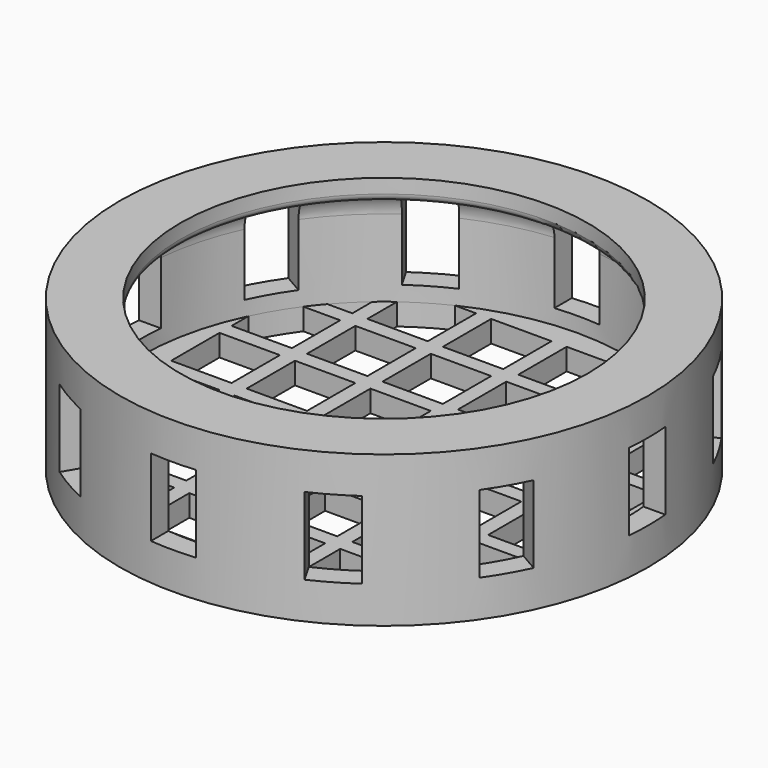
from build123d import *

# Parameters (mm, degrees)
F2_W            = 4
F2_H            = 4
F3_DEPTH        = 1.44
F4_R            = 17.5
F4_R_2          = 16.06
F5_DEPTH        = 1.44
F6_W            = 4
F6_H            = 5.12
F7_DEPTH        = 1.5
F7_COPIES_COUNT = 12


# Not quite as in the source:
# - a pattern or mirror of a feature is missing from the dataset's text; its kind, count and spacing are read off the source's solid


with BuildPart() as f1:
    # F0 (on Front) → F1 (revolve)
    with BuildSketch(Plane.XZ):
        with BuildLine():
            Line((0, 1.44), (0, 0))
            Line((0, 0), (17.5, 0))
            Line((17.5, 0), (17.5, 10))
            Line((17.5, 10), (13.5, 10))
            Line((13.5, 10), (13.5, 9.06))
            ThreePointArc((13.5, 9.06), (13.6464466094, 8.7064466094), (14, 8.56))
            Line((14, 8.56), (14.06, 8.56))
            ThreePointArc((14.06, 8.56), (15.4742135624, 7.9742135624), (16.06, 6.56))
            Line((16.06, 6.56), (16.06, 1.44))
            Line((16.06, 1.44), (0, 1.44))
        make_face()
    revolve(axis=Axis((0, 0, 0.72), (0, 0, 1)))

    # F2 (on face) → F3 (cut, through all)
    with BuildSketch(Plane(origin=(0, 0, 0), x_dir=(1, 0, 0), z_dir=(0, 0, -1))):
        with Locations((2.5, 2.5)):
            Rectangle(F2_W, F2_H)
        with Locations((2.5, 7.5)):
            Rectangle(F2_W, F2_H)
        with Locations((2.5, 12.5)):
            Rectangle(F2_W, F2_H)
        with Locations((7.5, 2.5)):
            Rectangle(F2_W, F2_H)
        with Locations((7.5, 7.5)):
            Rectangle(F2_W, F2_H)
        with Locations((7.5, 12.5)):
            Rectangle(F2_W, F2_H)
        with Locations((12.5, 2.5)):
            Rectangle(F2_W, F2_H)
        with Locations((12.5, 7.5)):
            Rectangle(F2_W, F2_H)
        with Locations((12.5, 12.5)):
            Rectangle(F2_W, F2_H)
        with Locations((-12.5, 2.5)):
            Rectangle(F2_W, F2_H)
        with Locations((-2.5, 2.5)):
            Rectangle(F2_W, F2_H)
        with Locations((-7.5, 7.5)):
            Rectangle(F2_W, F2_H)
        with Locations((-7.5, 12.5)):
            Rectangle(F2_W, F2_H)
        with Locations((-12.5, 7.5)):
            Rectangle(F2_W, F2_H)
        with Locations((-7.5, 2.5)):
            Rectangle(F2_W, F2_H)
        with Locations((-12.5, 12.5)):
            Rectangle(F2_W, F2_H)
        with Locations((-2.5, 7.5)):
            Rectangle(F2_W, F2_H)
        with Locations((-2.5, 12.5)):
            Rectangle(F2_W, F2_H)
        with Locations((2.5, -2.5)):
            Rectangle(F2_W, F2_H)
        with Locations((12.5, -2.5)):
            Rectangle(F2_W, F2_H)
        with Locations((-2.5, -2.5)):
            Rectangle(F2_W, F2_H)
        with Locations((-12.5, -7.5)):
            Rectangle(F2_W, F2_H)
        with Locations((-2.5, -12.5)):
            Rectangle(F2_W, F2_H)
        with Locations((12.5, -12.5)):
            Rectangle(F2_W, F2_H)
        with Locations((7.5, -12.5)):
            Rectangle(F2_W, F2_H)
        with Locations((7.5, -7.5)):
            Rectangle(F2_W, F2_H)
        with Locations((12.5, -7.5)):
            Rectangle(F2_W, F2_H)
        with Locations((-12.5, -2.5)):
            Rectangle(F2_W, F2_H)
        with Locations((-7.5, -2.5)):
            Rectangle(F2_W, F2_H)
        with Locations((-2.5, -7.5)):
            Rectangle(F2_W, F2_H)
        with Locations((-7.5, -12.5)):
            Rectangle(F2_W, F2_H)
        with Locations((7.5, -2.5)):
            Rectangle(F2_W, F2_H)
        with Locations((-7.5, -7.5)):
            Rectangle(F2_W, F2_H)
        with Locations((2.5, -12.5)):
            Rectangle(F2_W, F2_H)
        with Locations((2.5, -7.5)):
            Rectangle(F2_W, F2_H)
        with Locations((-12.5, -12.5)):
            Rectangle(F2_W, F2_H)
    extrude(amount=-F3_DEPTH, mode=Mode.SUBTRACT)

    # F4 (on face) → F5 (join, through all)
    with BuildSketch(Plane(origin=(0, 0, 0), x_dir=(1, 0, 0), z_dir=(0, 0, -1))):
        Circle(F4_R)
        Circle(F4_R_2, mode=Mode.SUBTRACT)
    extrude(amount=-F5_DEPTH)

    # F6 (on Front) → F7 (cut, symmetric)
    with BuildSketch(Plane.XZ):
        with Locations((15.5, 5)):
            Rectangle(F6_W, F6_H)
    f7 = extrude(amount=F7_DEPTH, both=True, mode=Mode.SUBTRACT)

    # F7_copies: F7 ×12 about axis
    f7_copies_axis = Axis((0, 0, 0), (0, 0, 1))
    for i in range(1, F7_COPIES_COUNT):
        add(f7.rotate(f7_copies_axis, i * 360 / F7_COPIES_COUNT), mode=Mode.SUBTRACT)


solid = f1.part
